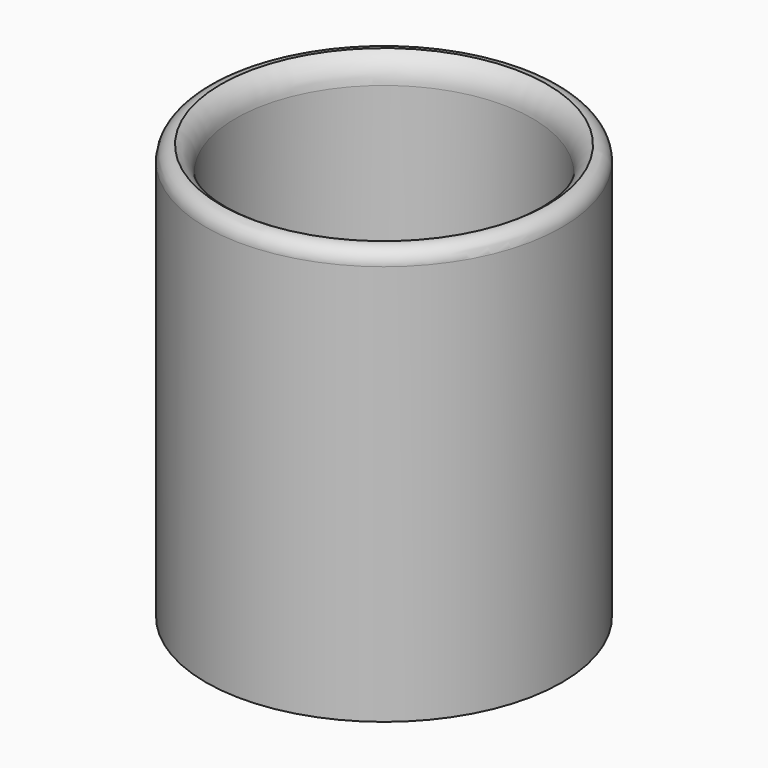
from build123d import *

# Parameters (mm, degrees)
F0_R     = 30
F0_R_2   = 25
F1_DEPTH = 70
F2_DEPTH = 7
F3_R     = 2.5


# Not quite as in the source:
# - a fillet or chamfer that OpenCascade refuses, or shapes differently, is made with other operations: its cross-section is extruded or revolved along the edge and cut away or added


with BuildPart() as f1:
    # F0 (on Top) → F1 (new body)
    with BuildSketch(Plane.XY):
        Circle(F0_R)
        Circle(F0_R_2, mode=Mode.SUBTRACT)
    extrude(amount=F1_DEPTH)

    # F0 (on Top) → F2 (join)
    with BuildSketch(Plane.XY):
        Circle(F0_R_2)
    extrude(amount=F2_DEPTH)

    # F3
    f3_edges = [f1.edges().sort_by_distance(p)[0] for p in [
        (-30, 0, 70),
    ]]
    fillet(f3_edges, radius=F3_R)

    # F4: fillet of radius 4.8284271247 on 1 edges, made by hand

    # F4_s1 → F4_t2 (revolve, cut)
    with BuildSketch(Plane.XZ):
        with BuildLine():
            ThreePointArc((27.5, 70), (25.6717247547, 68.2268227163), (25, 65.7700903528))
            Line((25, 65.7700903528), (24.9034314575, 65.7700903528))
            Line((24.9034314575, 65.7700903528), (24.9034314575, 70))
            Line((24.9034314575, 70), (25, 70.0965685425))
            ThreePointArc((25, 70.0965685425), (26.25, 70.0965685425), (27.4534314575, 70.0845981929))
            Line((27.4534314575, 70.0845981929), (27.5, 70))
        make_face()
    revolve(axis=Axis((0, 0, 70), (0, 0, 1)), mode=Mode.SUBTRACT)


solid = f1.part
